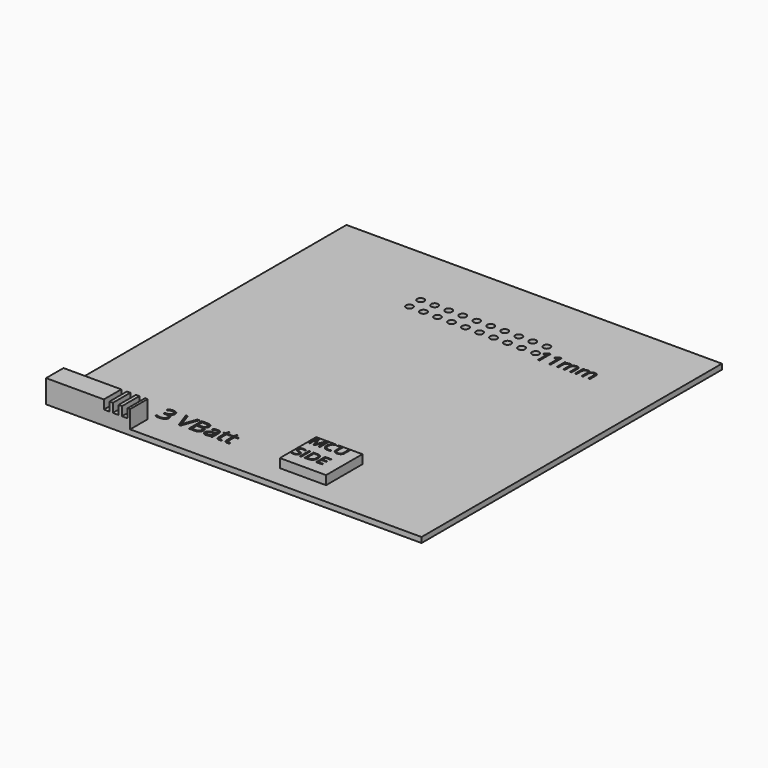
from build123d import *

# Parameters (mm, degrees)
F0_W            = 53.594
F0_H            = 53.594
F1_DEPTH        = 0.762
F2_R            = 0.5
F3_DEPTH        = 25.4
F4_W            = 12
F4_H            = 3.110745603
F5_DEPTH        = 2.54
F6_TEXT_SIZE    = 2.9225145323
F7_DEPTH        = 1.27
F8_W            = 6.5933982842
F8_H            = 6.4788423479
F9_DEPTH        = 1.27
F10_TEXT_SIZE   = 2.2721364176
F11_DEPTH       = 1.27
F12_W           = 8.5
F12_H           = 2.54
F13_DEPTH       = 2.54
F14_W           = 0.762
F14_H           = 2.54
F14_TEXT_SIZE   = 2.0340804816
F15_DEPTH       = 1.27
F17_DEPTH       = 0.254
F18_TEXT_SIZE   = 3.8717317188
F19_DEPTH       = 0.254
F20_W           = 0.8062236011
F20_H           = 3.110745603
F21_DEPTH       = 1.27
F22_TEXT_SIZE   = 3.2494853561
F23_DEPTH       = 0.254
F24_TEXT_SIZE   = 2.7945394524
F25_DEPTH       = 0.254
F26_TEXT_SIZE   = 1.5613504298
F26_TEXT_SIZE_2 = 2.7676811442
F27_DEPTH       = 0.254


# Not quite as in the source:
# - Text() gives the source's letters only with a copy of the font that has no kerning and outlines rounded to 1/6400 em; it was checked with that copy


with BuildPart() as f1:
    # F0 (on Top) → F1 (new body)
    with BuildSketch(Plane.XY):
        Rectangle(F0_W, F0_H)
    extrude(amount=F1_DEPTH)

    # F2 (on face) → F3 (cut)
    with BuildSketch(Plane.XY.offset(0.762)):
        with Locations((-8.9999996126, 15.797)):
            Circle(F2_R)
        with Locations((-8.9999996126, 17.797)):
            Circle(F2_R)
        with Locations((-6.9999996126, 15.797)):
            Circle(F2_R)
        with Locations((-6.9999996126, 17.797)):
            Circle(F2_R)
        with Locations((-4.9999996126, 15.797)):
            Circle(F2_R)
        with Locations((-4.9999996126, 17.797)):
            Circle(F2_R)
        with Locations((-2.9999996126, 15.797)):
            Circle(F2_R)
        with Locations((-2.9999996126, 17.797)):
            Circle(F2_R)
        with Locations((-0.9999996126, 15.797)):
            Circle(F2_R)
        with Locations((-0.9999996126, 17.797)):
            Circle(F2_R)
        with Locations((1.0000003874, 15.797)):
            Circle(F2_R)
        with Locations((1.0000003874, 17.797)):
            Circle(F2_R)
        with Locations((3.0000003874, 15.797)):
            Circle(F2_R)
        with Locations((3.0000003874, 17.797)):
            Circle(F2_R)
        with Locations((5.0000003874, 15.797)):
            Circle(F2_R)
        with Locations((5.0000003874, 17.797)):
            Circle(F2_R)
        with Locations((7.0000003874, 15.797)):
            Circle(F2_R)
        with Locations((7.0000003874, 17.797)):
            Circle(F2_R)
        with Locations((9.0000003874, 15.797)):
            Circle(F2_R)
        with Locations((9.0000003874, 17.797)):
            Circle(F2_R)
    extrude(amount=-F3_DEPTH, mode=Mode.SUBTRACT)

    # F4 (on face) → F5 (join)
    with BuildSketch(Plane.XY.offset(0.762)):
        with Locations((-20.797, -25.2416271985)):
            Rectangle(F4_W, F4_H)
    extrude(amount=F5_DEPTH)

    # F6 (on face) → F7 (cut)
    with BuildSketch(Plane.XY.offset(0.762)):
        with Locations((-26.0449081467, -22.860858892)):
            Text('24pin', F6_TEXT_SIZE, font='Open Sans', text_align=(TextAlign.LEFT, TextAlign.BOTTOM))
    extrude(amount=-F7_DEPTH, mode=Mode.SUBTRACT)

    # F8 (on face) → F9 (join)
    with BuildSketch(Plane.XY.offset(0.762)):
        with Locations((7.3816182659, -20.4468332231)):
            Rectangle(F8_W, F8_H)
    extrude(amount=F9_DEPTH)

    # F10 (on face) → F11 (cut)
    with BuildSketch(Plane.XY.offset(2.032)):
        with Locations((4.0849191238, -18.8433502699)):
            Text('MCU', F10_TEXT_SIZE, font='Open Sans', text_align=(TextAlign.LEFT, TextAlign.BOTTOM))
        with Locations((4.0849191238, -21.9334557979)):
            Text('SIDE', F10_TEXT_SIZE, font='Open Sans', text_align=(TextAlign.LEFT, TextAlign.BOTTOM))
    extrude(amount=-F11_DEPTH, mode=Mode.SUBTRACT)

    # F12 (on face) → F13 (join)
    with BuildSketch(Plane(origin=(0, 0, 0), x_dir=(1, 0, 0), z_dir=(0, 0, -1))):
        with Locations((-8.5, 5.527)):
            Rectangle(F12_W, F12_H)
    extrude(amount=F13_DEPTH)

    # F14 (on face) → F15 (cut)
    with BuildSketch(Plane(origin=(0, 0, -2.54), x_dir=(1, 0, 0), z_dir=(0, 0, -1))):
        with Locations((-12.0971467021, 5.527)):
            Rectangle(F14_W, F14_H)
        with Locations((-10.9534195018, 5.527)):
            Rectangle(F14_W, F14_H)
        with Locations(Location((-4.25, 6.797), (0, 0, -180))):
            Text('16 Pin', F14_TEXT_SIZE, font='Open Sans', text_align=(TextAlign.LEFT, TextAlign.BOTTOM))
    extrude(amount=-F15_DEPTH, mode=Mode.SUBTRACT)

    # F16 (on face) → F17 (cut)
    with BuildSketch(Plane(origin=(0, 0, 0), x_dir=(1, 0, 0), z_dir=(0, 0, -1))):
        Polygon((-7.9473047987, 6.797), (-7.9473047987, 8.6307629735), (-6.8091066093, 8.6307629735), (-8.4524019621, 11.1600907312), (-10.3493984789, 8.6307629735), (-9.2112002894, 8.6307629735), (-9.2112002894, 6.797), align=None)
    extrude(amount=-F17_DEPTH, mode=Mode.SUBTRACT)

    # F18 (on face) → F19 (cut)
    with BuildSketch(Plane(origin=(0, 0, 0), x_dir=(1, 0, 0), z_dir=(0, 0, -1))):
        with Locations(Location((-12.1059147641, 10.2338844445), (0, 0, 180))):
            Text('2 GNDs', F18_TEXT_SIZE, font='Open Sans', text_align=(TextAlign.LEFT, TextAlign.BOTTOM))
    extrude(amount=-F19_DEPTH, mode=Mode.SUBTRACT)

    # F20 (on face) → F21 (cut)
    with BuildSketch(Plane.XY.offset(3.302)):
        with Locations((-15.5580304563, -25.2416271985)):
            Rectangle(F20_W, F20_H)
        with Locations((-16.8543104082, -25.2416271985)):
            Rectangle(F20_W, F20_H)
        with Locations((-18.1505903602, -25.2416271985)):
            Rectangle(F20_W, F20_H)
    extrude(amount=-F21_DEPTH, mode=Mode.SUBTRACT)

    # F22 (on face) → F23 (cut)
    with BuildSketch(Plane.XY.offset(0.762)):
        with Locations((-14.7714670748, -22.5770175457)):
            Text('3 VBatt', F22_TEXT_SIZE, font='Open Sans', text_align=(TextAlign.LEFT, TextAlign.BOTTOM))
    extrude(amount=-F23_DEPTH, mode=Mode.SUBTRACT)

    # F24 (on face) → F25 (cut)
    with BuildSketch(Plane.XY.offset(0.762)):
        with Locations((9.4684287906, 14.6852778271)):
            Text('11mm', F24_TEXT_SIZE, font='Open Sans', text_align=(TextAlign.LEFT, TextAlign.BOTTOM))
    extrude(amount=-F25_DEPTH, mode=Mode.SUBTRACT)

    # F26 (on face) → F27 (cut)
    with BuildSketch(Plane(origin=(0, 0, 0), x_dir=(1, 0, 0), z_dir=(0, 0, -1))):
        with Locations(Location((-5.96, 4.257), (0, 0, 180))):
            Text('8.5mm', F26_TEXT_SIZE, font='Open Sans', text_align=(TextAlign.LEFT, TextAlign.BOTTOM))
        with Locations(Location((-5.9076010366, 15.586397436), (0, 0, -90))):
            Text('20mm', F26_TEXT_SIZE_2, font='Open Sans', text_align=(TextAlign.LEFT, TextAlign.BOTTOM))
    extrude(amount=-F27_DEPTH, mode=Mode.SUBTRACT)


solid = f1.part
